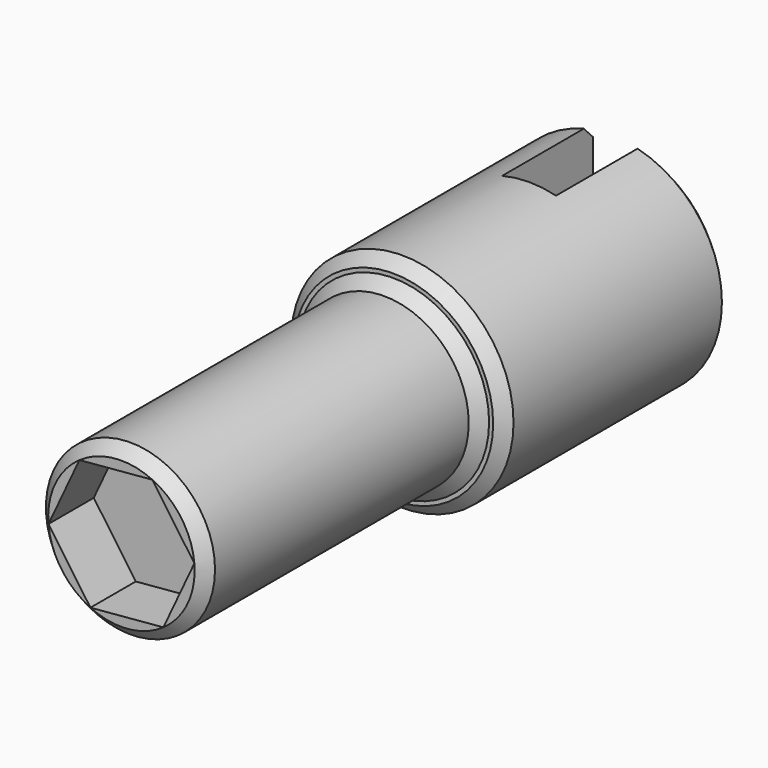
from build123d import *

# Parameters (mm, degrees)
F0_R      = 49.9014426293
F1_DEPTH  = 127
F2_R      = 37.9248906149
F3_DEPTH  = 152.4
F4_SIZE   = 5.08
F6_DEPTH  = 25.4
F9_W      = 24.138873443
F9_H      = 129.7791451216
F10_DEPTH = 50.8


# Not quite as in the source:
# - the program builds the solid bodies; features that only make, move or delete a surface that nothing else refers to are left out


with BuildPart() as f1:
    # F0 (on Front) → F1 (new body)
    with BuildSketch(Plane.XZ):
        Circle(F0_R)
    extrude(amount=F1_DEPTH)

    # F2 (on face) → F3 (join)
    with BuildSketch(Plane.XZ.offset(127)):
        Circle(F2_R)
    extrude(amount=F3_DEPTH)

    # F4
    f4_edges = [f1.edges().sort_by_distance(p)[0] for p in [
        (-49.901443, -127, 0),
        (-37.924891, -127, 0),
        (-37.924891, -279.4, 0),
        (-49.901443, 0, 0),
    ]]
    chamfer(f4_edges, length=F4_SIZE)

    # F5 (on face) → F6 (cut)
    with BuildSketch(Plane.XZ.offset(279.4)):
        Polygon((-13.8807385989, -29.7676323455), (18.8391565222, -26.9048884227), (32.7198951211, 2.8627439228), (13.8807385989, 29.7676323455), (-18.8391565222, 26.9048884227), (-32.7198951211, -2.8627439228), align=None)
    extrude(amount=-F6_DEPTH, mode=Mode.SUBTRACT)

    # F9 (on face) → F10 (cut)
    with BuildSketch(Plane(origin=(0, 0, 0), x_dir=(-1, 0, 0), z_dir=(0, 1, 0))):
        Rectangle(F9_W, F9_H)
    extrude(amount=-F10_DEPTH, mode=Mode.SUBTRACT)


solid = f1.part
